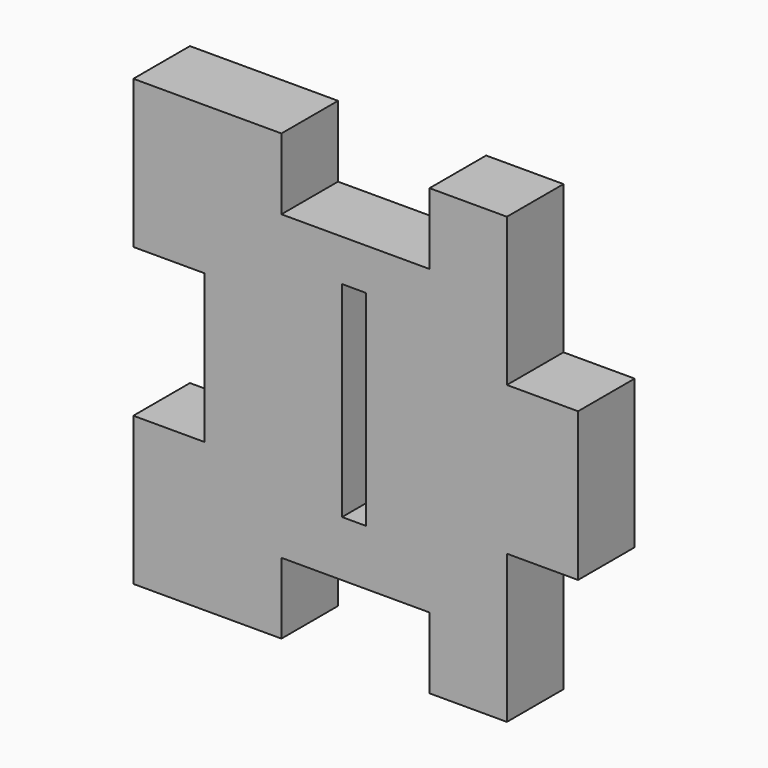
from build123d import *

# Parameters (mm, degrees)
F1_DEPTH     = 2.032
F2_TEXT_SIZE = 8.2535277778
F3_DEPTH     = 1


# Not quite as in the source:
# - a length typed as a fraction of an inch, garbled in the dataset ("3 / 203.2 mm" for 3/8 in), is restored
# - Text() gives the source's letters only with a copy of the font that has no kerning and outlines rounded to 1/6400 em; it was checked with that copy


with BuildPart() as f1:
    # F0 (on Front) → F1 (new body)
    with BuildSketch(Plane.XZ):
        Polygon((-10.9897290399, 29.0234165891), (-10.9897290399, 26.8898165891), (-10.9897290399, 24.7562165891), (-13.0344290399, 24.7562165891), (-13.0344290399, 20.5017165891), (-8.7799290399, 20.5017165891), (-8.7799290399, 22.5464165891), (-4.5254290399, 22.5464165891), (-4.5254290399, 20.5017165891), (-2.3029290399, 20.5017165891), (-2.3029290399, 24.7562165891), (-0.2582290399, 24.7562165891), (-0.2582290399, 29.0234165891), (-2.3029290399, 29.0234165891), (-2.3029290399, 33.2779165891), (-4.5254290399, 33.2779165891), (-4.5254290399, 31.2332165891), (-8.7799290399, 31.2332165891), (-8.7799290399, 33.2779165891), (-13.0344290399, 33.2779165891), (-13.0344290399, 29.0234165891), align=None)
    extrude(amount=F1_DEPTH)

    # F2 (on face) → F3 (cut)
    with BuildSketch(Plane.XZ.offset(2.032)):
        with Locations((-7.8484847465, 24.1429156834)):
            Text('I', F2_TEXT_SIZE, font='Open Sans', text_align=(TextAlign.LEFT, TextAlign.BOTTOM))
    extrude(amount=-F3_DEPTH, mode=Mode.SUBTRACT)


solid = f1.part
